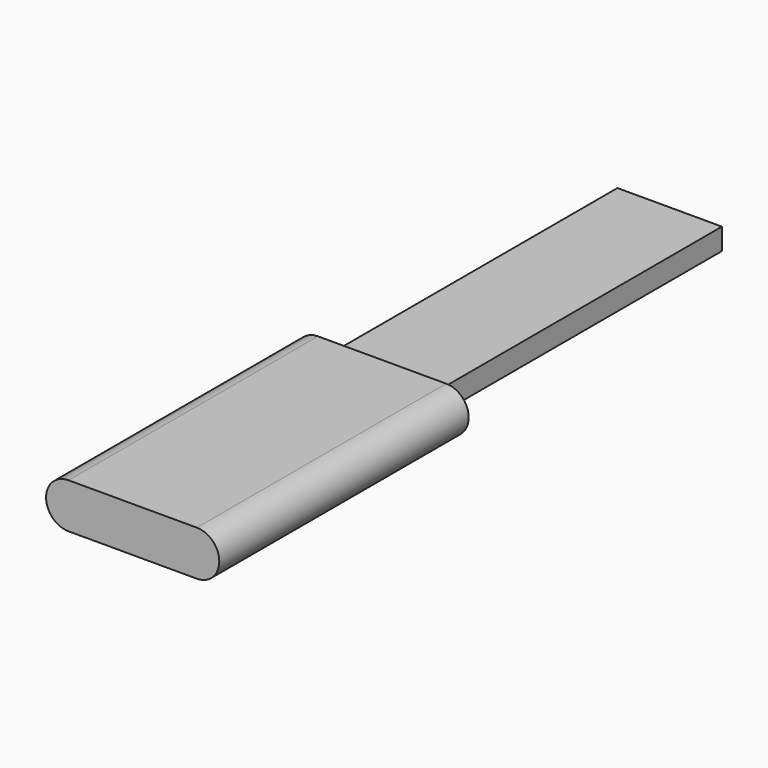
from build123d import *

# Parameters (mm, degrees)
F1_DEPTH = 254
F2_W     = 85.141710937
F2_H     = 17.5291653723
F3_DEPTH = 292.8777724


# Not quite as in the source:
# - an extrude ends at something that could not be found from the text; its depth is read off the source's solid


with BuildPart() as f1:
    # F0 (on Front) → F1 (new body)
    with BuildSketch(Plane.XZ):
        with BuildLine():
            Line((52.2444248199, 18.3139387518), (-52.2444248199, 18.3139387518))
            ThreePointArc((-52.2444248199, 18.3139387518), (-70.5583635718, 0), (-52.2444248199, -18.3139387518))
            Line((-52.2444248199, -18.3139387518), (52.2444248199, -18.3139387518))
            ThreePointArc((52.2444248199, -18.3139387518), (70.5583635718, 0), (52.2444248199, 18.3139387518))
        make_face()
    extrude(amount=F1_DEPTH)

    # F2 (on Front) → F3 (join, through all)
    with BuildSketch(Plane.XZ):
        Rectangle(F2_W, F2_H)
    extrude(amount=-F3_DEPTH)


solid = f1.part
